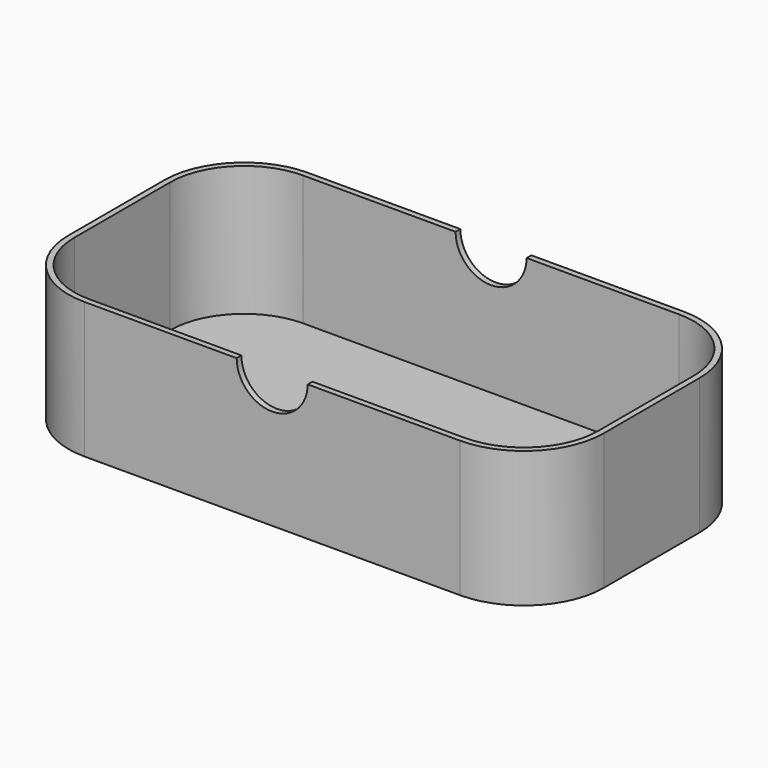
from build123d import *

# Parameters (mm, degrees)
F0_W     = 181
F0_H     = 94.5
F1_DEPTH = 46
F2_R     = 27
F3_T     = -2
F4_R     = 12
F5_DEPTH = 105


with BuildPart() as f1:
    # F0 (on Top) → F1 (new body)
    with BuildSketch(Plane.XY):
        with Locations((-9.7413412556, -21.9173085093)):
            Rectangle(F0_W, F0_H)
    extrude(amount=-F1_DEPTH)

    # F2
    f2_edges = [f1.edges().sort_by_distance(p)[0] for p in [
        (80.758659, 25.332691, -23),
        (-100.241341, 25.332691, -23),
        (-100.241341, -69.167309, -23),
        (80.758659, -69.167309, -23),
    ]]
    fillet(f2_edges, radius=F2_R)

    # F3
    f3_openings = [f1.faces().sort_by_distance(p)[0] for p in [
        (-9.741341, -21.917309, 0),
    ]]
    offset(amount=F3_T, openings=f3_openings)

    # F4 (on face) → F5 (cut)
    with BuildSketch(Plane.XZ.offset(69.1673085093)):
        with Locations((-9.7413412556, 0)):
            Circle(F4_R)
    extrude(amount=-F5_DEPTH, mode=Mode.SUBTRACT)


solid = f1.part
